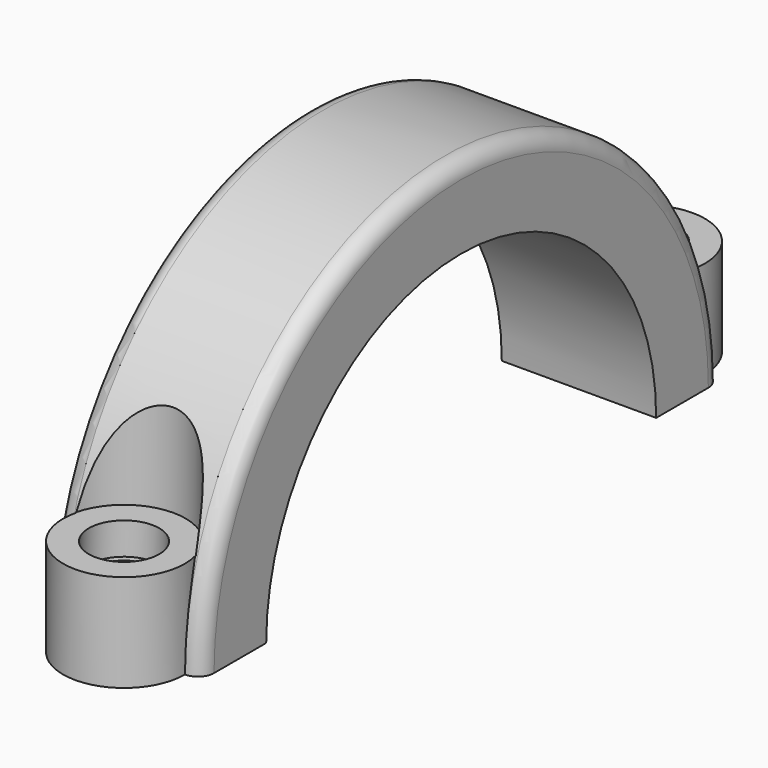
from build123d import *

# Parameters (mm, degrees)
F1_DEPTH       = 12.065
F2_R           = 9.525
F3_DEPTH       = 15.25
F4_R           = 9.625
F5_DEPTH       = 25
F7_D           = 9
F7_DEPTH       = 75
F7_CBORE_D     = 11
F7_CBORE_DEPTH = 5
F7_TIP         = 2.7038727856
F8_R           = 2.5


# Not quite as in the source:
# - a pattern or mirror of a feature is missing from the dataset's text; its kind, count and spacing are read off the source's solid


with BuildPart() as f1:
    # F0 (on Right) → F1 (new body, symmetric)
    with BuildSketch(Plane.YZ):
        with BuildLine():
            ThreePointArc((-38.1, 0), (0, 38.1), (38.1, 0))
            Line((38.1, 0), (50.8, 0))
            ThreePointArc((50.8, 0), (0, 50.8), (-50.8, 0))
            Line((-50.8, 0), (-38.1, 0))
        make_face()
    extrude(amount=F1_DEPTH, both=True)

    # F2 (on face) → F3 (join)
    with BuildSketch(Plane(origin=(0, 0, 0), x_dir=(1, 0, 0), z_dir=(0, 0, -1))):
        with Locations((0, -50.8)):
            Circle(F2_R)
    f3 = extrude(amount=-F3_DEPTH)

    # F3_copies: F3 across plane
    add(f3.mirror(Plane(origin=(0, 0, 0), x_dir=(0, 0, -1), z_dir=(0, -1, 0))))

    # F4 (on face) → F5 (cut)
    with BuildSketch(Plane.XY.offset(15.25)):
        with Locations((0, 50.8)):
            Circle(F4_R)
    f5 = extrude(amount=F5_DEPTH, mode=Mode.SUBTRACT)

    # F5_copies: F5 across plane
    add(f5.mirror(Plane(origin=(0, -4e-06, 0), x_dir=(0, 0, -1), z_dir=(0, -1, 0))), mode=Mode.SUBTRACT)

    # F7
    with Locations(Plane.XY.offset(15.25)):
        with Locations((0, 50.8)):
            f7 = CounterBoreHole(F7_D / 2, F7_CBORE_D / 2, F7_CBORE_DEPTH, depth=F7_DEPTH)
            with Locations((0, 0, -(F7_DEPTH + F7_TIP / 2))):  # 118° drill point
                Cone(0, F7_D / 2, F7_TIP, mode=Mode.SUBTRACT)

    # F7_copies: F7 across plane
    add(f7.mirror(Plane(origin=(0, 0, 0), x_dir=(0, 0, -1), z_dir=(0, -1, 0))), mode=Mode.SUBTRACT)

    # F8
    f8_edges = [f1.edges().sort_by_distance(p)[0] for p in [
        (12.065, 0, 50.8),
        (-12.065, 0, 50.8),
    ]]
    fillet(f8_edges, radius=F8_R)


solid = f1.part
